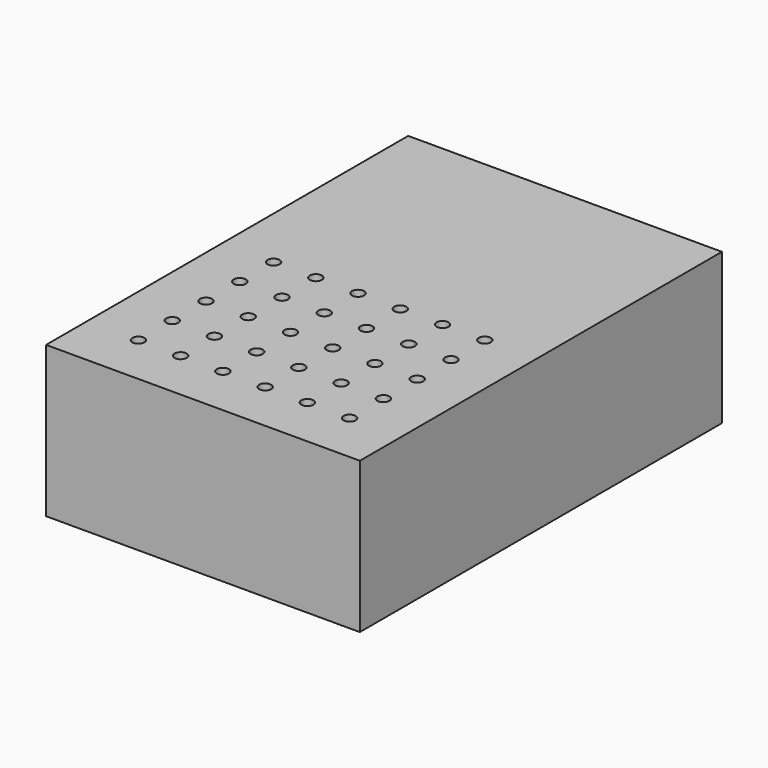
from build123d import *

# Parameters (mm, degrees)
F0_W     = 104
F0_H     = 150
F0_R     = 2
F1_DEPTH = 50
F2_T     = -5
F3_DEPTH = 25


# Not quite as in the source:
# - a feature names something its author has since deleted; it is built from what else it names


with BuildPart() as f1:
    # F0 (on Top) → F1 (new body)
    with BuildSketch(Plane.XY):
        with Locations((0, 30)):
            Rectangle(F0_W, F0_H)
        with Locations((-35, -28)):
            Circle(F0_R, mode=Mode.SUBTRACT)
        with Locations((-35, -14)):
            Circle(F0_R, mode=Mode.SUBTRACT)
        with Locations((-21, -28)):
            Circle(F0_R, mode=Mode.SUBTRACT)
        with Locations((-7, -28)):
            Circle(F0_R, mode=Mode.SUBTRACT)
        with Locations((-21, -14)):
            Circle(F0_R, mode=Mode.SUBTRACT)
        with Locations((-7, -14)):
            Circle(F0_R, mode=Mode.SUBTRACT)
        with Locations((-35, 0)):
            Circle(F0_R, mode=Mode.SUBTRACT)
        with Locations((-35, 14)):
            Circle(F0_R, mode=Mode.SUBTRACT)
        with Locations((-35, 28)):
            Circle(F0_R, mode=Mode.SUBTRACT)
        with Locations((-21, 0)):
            Circle(F0_R, mode=Mode.SUBTRACT)
        with Locations((-7, 0)):
            Circle(F0_R, mode=Mode.SUBTRACT)
        with Locations((-21, 14)):
            Circle(F0_R, mode=Mode.SUBTRACT)
        with Locations((-21, 28)):
            Circle(F0_R, mode=Mode.SUBTRACT)
        with Locations((-7, 14)):
            Circle(F0_R, mode=Mode.SUBTRACT)
        with Locations((-7, 28)):
            Circle(F0_R, mode=Mode.SUBTRACT)
        with Locations((7, -28)):
            Circle(F0_R, mode=Mode.SUBTRACT)
        with Locations((21, -28)):
            Circle(F0_R, mode=Mode.SUBTRACT)
        with Locations((7, -14)):
            Circle(F0_R, mode=Mode.SUBTRACT)
        with Locations((21, -14)):
            Circle(F0_R, mode=Mode.SUBTRACT)
        with Locations((35, -28)):
            Circle(F0_R, mode=Mode.SUBTRACT)
        with Locations((35, -14)):
            Circle(F0_R, mode=Mode.SUBTRACT)
        with Locations((7, 0)):
            Circle(F0_R, mode=Mode.SUBTRACT)
        with Locations((21, 0)):
            Circle(F0_R, mode=Mode.SUBTRACT)
        with Locations((7, 14)):
            Circle(F0_R, mode=Mode.SUBTRACT)
        with Locations((7, 28)):
            Circle(F0_R, mode=Mode.SUBTRACT)
        with Locations((21, 14)):
            Circle(F0_R, mode=Mode.SUBTRACT)
        with Locations((21, 28)):
            Circle(F0_R, mode=Mode.SUBTRACT)
        with Locations((35, 0)):
            Circle(F0_R, mode=Mode.SUBTRACT)
        with Locations((35, 14)):
            Circle(F0_R, mode=Mode.SUBTRACT)
        with Locations((35, 28)):
            Circle(F0_R, mode=Mode.SUBTRACT)
        with Locations((7, -28)):
            Circle(F0_R)
        with Locations((35, 14)):
            Circle(F0_R)
        with Locations((21, 0)):
            Circle(F0_R)
        with Locations((21, 28)):
            Circle(F0_R)
        with Locations((7, 28)):
            Circle(F0_R)
        with Locations((35, -28)):
            Circle(F0_R)
        with Locations((-7, -14)):
            Circle(F0_R)
        with Locations((-7, -28)):
            Circle(F0_R)
        with Locations((7, 14)):
            Circle(F0_R)
        with Locations((-35, 28)):
            Circle(F0_R)
        with Locations((-35, 14)):
            Circle(F0_R)
        with Locations((-35, 0)):
            Circle(F0_R)
        with Locations((-35, -14)):
            Circle(F0_R)
        with Locations((-35, -28)):
            Circle(F0_R)
        with Locations((-21, 28)):
            Circle(F0_R)
        with Locations((-21, 14)):
            Circle(F0_R)
        with Locations((-21, 0)):
            Circle(F0_R)
        with Locations((-21, -14)):
            Circle(F0_R)
        with Locations((-21, -28)):
            Circle(F0_R)
        with Locations((-7, 28)):
            Circle(F0_R)
        with Locations((-7, 14)):
            Circle(F0_R)
        with Locations((-7, 0)):
            Circle(F0_R)
        with Locations((35, 0)):
            Circle(F0_R)
        with Locations((21, -14)):
            Circle(F0_R)
        with Locations((21, 14)):
            Circle(F0_R)
        with Locations((7, 0)):
            Circle(F0_R)
        with Locations((35, -14)):
            Circle(F0_R)
        with Locations((21, -28)):
            Circle(F0_R)
        with Locations((7, -14)):
            Circle(F0_R)
        with Locations((35, 28)):
            Circle(F0_R)
    extrude(amount=-F1_DEPTH)

    # F2
    f2_openings = [f1.faces().sort_by_distance(p)[0] for p in [
        (0, 30, -50),
    ]]
    offset(amount=F2_T, openings=f2_openings)

    # F0 (on Top) → F3 (cut)
    with BuildSketch(Plane.XY):
        with Locations((7, -14)):
            Circle(F0_R)
        with Locations((35, -14)):
            Circle(F0_R)
        with Locations((21, -28)):
            Circle(F0_R)
        with Locations((7, 0)):
            Circle(F0_R)
        with Locations((21, 14)):
            Circle(F0_R)
        with Locations((21, -14)):
            Circle(F0_R)
        with Locations((35, 0)):
            Circle(F0_R)
        with Locations((-7, 0)):
            Circle(F0_R)
        with Locations((-7, 14)):
            Circle(F0_R)
        with Locations((-7, 28)):
            Circle(F0_R)
        with Locations((-21, -28)):
            Circle(F0_R)
        with Locations((-21, -14)):
            Circle(F0_R)
        with Locations((-21, 0)):
            Circle(F0_R)
        with Locations((-21, 14)):
            Circle(F0_R)
        with Locations((-35, -28)):
            Circle(F0_R)
        with Locations((-35, -14)):
            Circle(F0_R)
        with Locations((-35, 0)):
            Circle(F0_R)
        with Locations((7, 14)):
            Circle(F0_R)
        with Locations((-7, -28)):
            Circle(F0_R)
        with Locations((-7, -14)):
            Circle(F0_R)
        with Locations((7, 28)):
            Circle(F0_R)
        with Locations((35, -28)):
            Circle(F0_R)
        with Locations((21, 28)):
            Circle(F0_R)
        with Locations((21, 0)):
            Circle(F0_R)
        with Locations((35, 14)):
            Circle(F0_R)
        with Locations((7, -28)):
            Circle(F0_R)
        with Locations((35, 28)):
            Circle(F0_R)
        with Locations((-21, 28)):
            Circle(F0_R)
        with Locations((-35, 14)):
            Circle(F0_R)
        with Locations((-35, 28)):
            Circle(F0_R)
    extrude(amount=-F3_DEPTH, mode=Mode.SUBTRACT)


solid = f1.part
